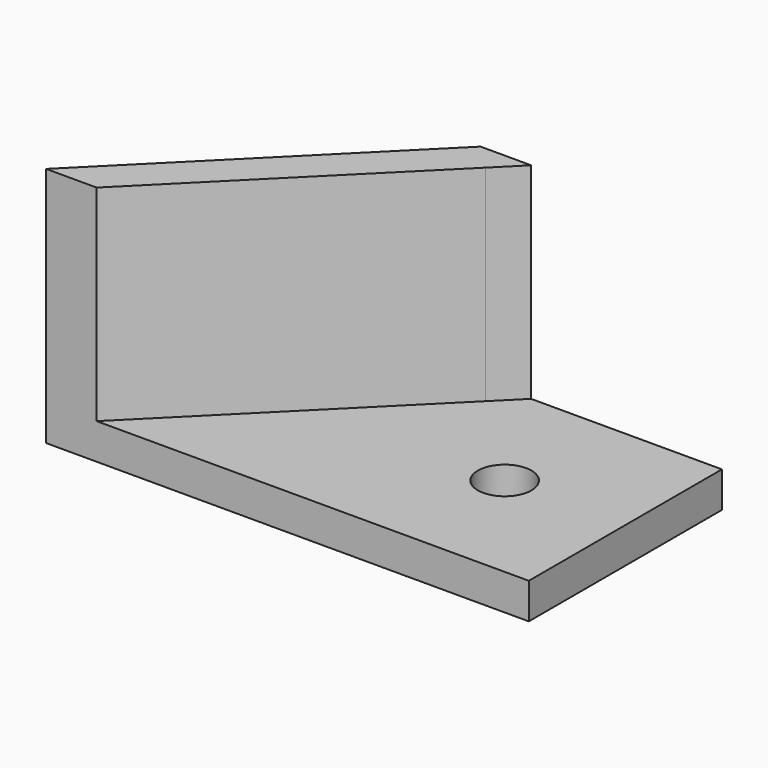
from build123d import *

# Parameters (mm, degrees)
F0_W     = 21.43125
F0_H     = 21.43125
F0_R     = 2.38125
F1_DEPTH = 3.175
F3_DEPTH = 18.25625


# Not quite as in the source:
# - a length typed as a fraction of an inch, garbled in the dataset ("3 / 203.2 mm" for 3/8 in), is restored


with BuildPart() as f1:
    # F0 (on Top) → F1 (new body)
    with BuildSketch(Plane.XY):
        Rectangle(F0_W, F0_H)
        Circle(F0_R, mode=Mode.SUBTRACT)
        Polygon((-10.715625, -10.715625), (-10.715625, 10.715625), (-32.146875, -10.715625), align=None)
    extrude(amount=F1_DEPTH)

    # F2 (on face) → F3 (join)
    with BuildSketch(Plane.XY.offset(3.175)):
        Polygon((-27.6567469395, -10.715625), (-8.4705609697, 8.4705609697), (-6.2254969395, 10.715625), (-10.715625, 10.715625), (-32.146875, -10.715625), align=None)
    extrude(amount=F3_DEPTH)


solid = f1.part
